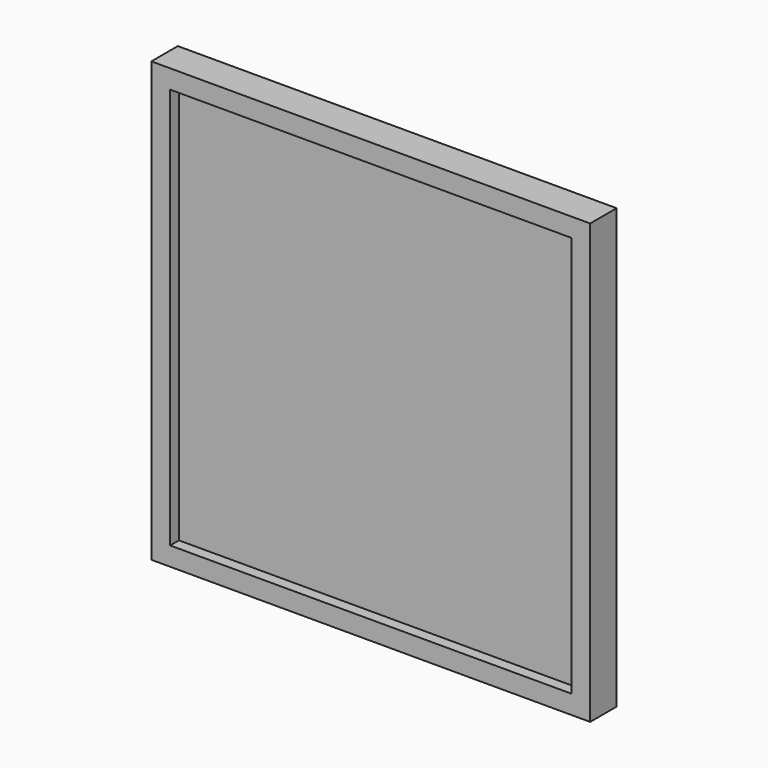
from build123d import *

# Parameters (mm, degrees)
F0_W     = 101.0093018413
F0_H     = 101.0093018413
F1_DEPTH = 5.08
F2_W     = 101.0093018413
F2_H     = 101.0093018413
F2_W_2   = 92.3733018413
F2_H_2   = 92.3733018413
F3_DEPTH = 2.54


# Not quite as in the source:
# - the program builds the solid bodies; features that only make, move or delete a surface that nothing else refers to are left out


with BuildPart() as f1:
    # F0 (on Front) → F1 (new body)
    with BuildSketch(Plane.XZ):
        Rectangle(F0_W, F0_H)
    extrude(amount=F1_DEPTH)

    # F2 (on face) → F3 (join)
    with BuildSketch(Plane.XZ.offset(5.08)):
        Rectangle(F2_W, F2_H)
        Rectangle(F2_W_2, F2_H_2, mode=Mode.SUBTRACT)
    extrude(amount=F3_DEPTH)


solid = f1.part
